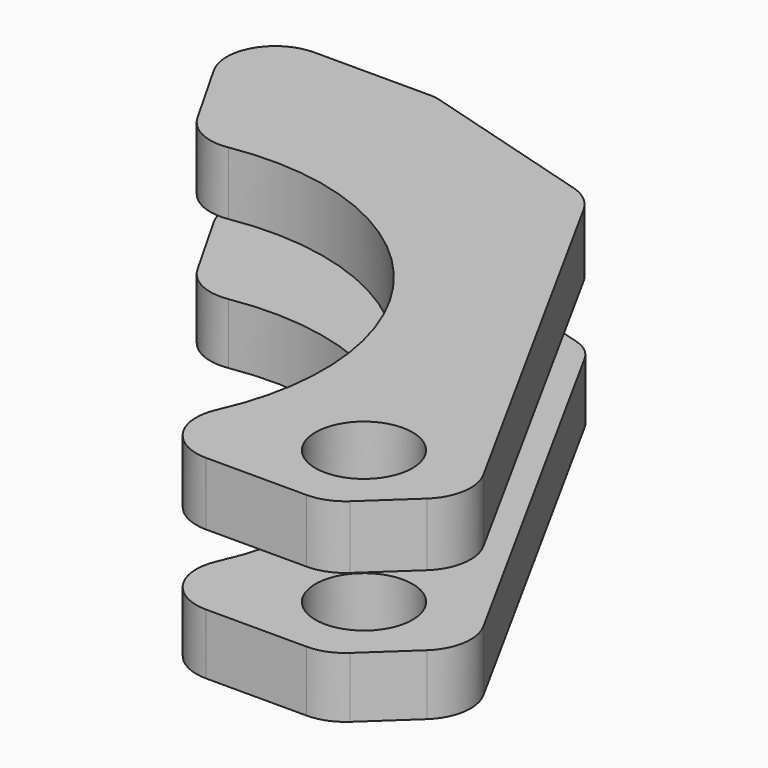
from build123d import *

# Parameters (mm, degrees)
F0_R        = 6.35
F1_DEPTH    = 25.4
F2_W        = 123.3146692741
F2_H        = 9.2131719061
F3_DEPTH    = 44.45
F4_R        = 6.35
F5_R        = 5.08
F6_R        = 5.08
F7_R        = 6.35
F8_R        = 6.35
F9_T1_DEPTH = 31.6918409034
F9_T3_DEPTH = 32.0036689973
F9_T5_DEPTH = 79.9823917725


# Not quite as in the source:
# - a fillet or chamfer that OpenCascade refuses, or shapes differently, is made with other operations: its cross-section is extruded or revolved along the edge and cut away or added


with BuildPart() as f1:
    # F0 (on Top) → F1 (new body)
    with BuildSketch(Plane.XY):
        with BuildLine():
            Line((-38.4631145681, 47.8382077998), (-25.4427038645, 24.9439910361))
            ThreePointArc((-25.4427038645, 24.9439910361), (12.1724359017, 10.8562296523), (7.9763394945, -29.0906918233))
            Line((7.9763394945, -29.0906918233), (35.5361980368, -29.0906918233))
            Line((35.5361980368, -29.0906918233), (46.7120397772, -18.6743740407))
            Line((46.7120397772, -18.6743740407), (14.3780414237, 40.2429682227))
            Line((14.3780414237, 40.2429682227), (-11.6627799835, 47.8382077998))
            Line((-11.6627799835, 47.8382077998), (-38.4631145681, 47.8382077998))
        make_face()
        with Locations((31.4130679807, -17.697843238)):
            Circle(F0_R, mode=Mode.SUBTRACT)
    extrude(amount=F1_DEPTH)

    # F2 (on Front) → F3 (cut, symmetric)
    with BuildSketch(Plane.XZ):
        with Locations((5.399286747, 12.5440859531)):
            Rectangle(F2_W, F2_H)
    extrude(amount=F3_DEPTH, both=True, mode=Mode.SUBTRACT)

    # F4
    f4_edges = [f1.edges().sort_by_distance(p)[0] for p in [
        (14.378041, 40.242968, 21.275336),
    ]]
    fillet(f4_edges, radius=F4_R)

    # F5
    f5_edges = [f1.edges().sort_by_distance(p)[0] for p in [
        (14.378041, 40.242968, 3.96875),
    ]]
    fillet(f5_edges, radius=F5_R)

    # F6
    f6_edges = [f1.edges().sort_by_distance(p)[0] for p in [
        (-11.66278, 47.838208, 12.7),
    ]]
    fillet(f6_edges, radius=F6_R)

    # F7
    f7_edges = [f1.edges().sort_by_distance(p)[0] for p in [
        (7.976339, -29.090692, 21.275336),
        (7.976339, -29.090692, 3.96875),
    ]]
    fillet(f7_edges, radius=F7_R)

    # F8
    f8_edges = [f1.edges().sort_by_distance(p)[0] for p in [
        (35.536198, -29.090692, 3.96875),
        (35.536198, -29.090692, 21.275336),
        (46.71204, -18.674374, 21.275336),
        (46.71204, -18.674374, 3.96875),
    ]]
    fillet(f8_edges, radius=F8_R)

    # F9: fillet of radius 6.35 on 3 edges, made by hand

    # F9_s2 → F9_t1 (cut)
    with BuildSketch(Plane.XY.offset(-11.8771704517)):
        with BuildLine():
            ThreePointArc((-21.2123797216, 25.95187937), (-24.9938313602, 26.4760275688), (-27.791358986, 29.0737086524))
            Line((-27.791358986, 29.0737086524), (-25.4427038645, 24.9439910361))
            ThreePointArc((-25.4427038645, 24.9439910361), (-23.3442549108, 25.5180837534), (-21.2123797216, 25.95187937))
        make_face()
    extrude(amount=F9_T1_DEPTH, mode=Mode.SUBTRACT)

    # F9_s4 → F9_t3 (cut)
    with BuildSketch(Plane.XY.offset(5.2735014544)):
        with BuildLine():
            ThreePointArc((-27.791358986, 29.0737086524), (-24.9938313602, 26.4760275688), (-21.2123797216, 25.95187937))
            ThreePointArc((-21.2123797216, 25.95187937), (-23.3442549108, 25.5180837534), (-25.4427038645, 24.9439910361))
            Line((-25.4427038645, 24.9439910361), (-27.791358986, 29.0737086524))
        make_face()
    extrude(amount=F9_T3_DEPTH, mode=Mode.SUBTRACT)

    # F9_s6 → F9_t5 (cut)
    with BuildSketch(Plane.XY.offset(-27.2911958862)):
        with BuildLine():
            ThreePointArc((-33.0664077304, 38.3490005109), (-33.0355553369, 44.6810539999), (-27.5466362136, 47.8382077998))
            Line((-27.5466362136, 47.8382077998), (-38.4631145681, 47.8382077998))
            Line((-38.4631145681, 47.8382077998), (-33.0664077304, 38.3490005109))
        make_face()
    extrude(amount=F9_T5_DEPTH, mode=Mode.SUBTRACT)


solid = f1.part
